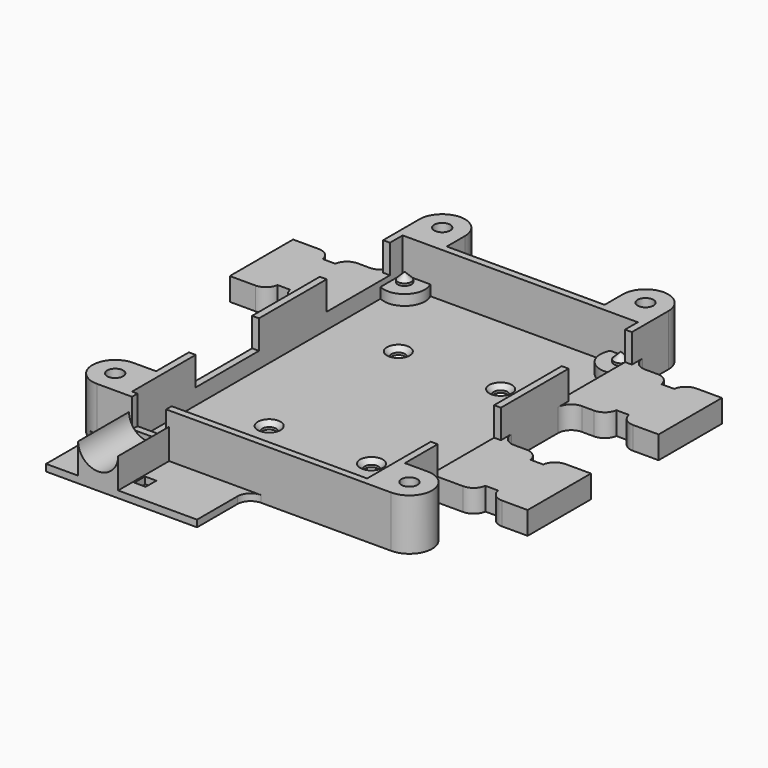
from build123d import *

# Parameters (mm, degrees)
F1_W          = 54.708
F1_H          = 77.4
F2_DEPTH      = 11.3
F3_T          = -1.5
F4_W          = 20.1
F4_H          = 17.4
F5_DEPTH      = 6.3
F6_R          = 4.5
F7_DEPTH      = 2.3
F8_R          = 1.5
F9_DEPTH      = 11.301
F10_SIZE      = 1
F11_R         = 1.75
F12_DEPTH     = 11.3
F13_R         = 1.5
F14_DEPTH     = 2
F15_SIZE      = 1.5
F16_W         = 7.5
F16_H         = 1.5
F17_DEPTH     = 6.3
F18_W         = 19.8
F18_H         = 17.4
F19_DEPTH     = 5
F20_W         = 33.2
F20_H         = 14
F21_DEPTH     = 1.5
F23_DEPTH     = 14
F24_W         = 2.5
F24_H         = 2.8
F24_W_2       = 2.8
F24_H_2       = 2.5
F24_W_3       = 2.5000000001
F24_H_3       = 2.940192353
F25_DEPTH     = 11.301
F26_T1_DEPTH  = 1.5
F26_T3_DEPTH  = 1.5
F26_T5_DEPTH  = 5
F26_T7_DEPTH  = 5
F26_T9_DEPTH  = 5
F26_T11_DEPTH = 5
F26_T13_DEPTH = 5
F26_T15_DEPTH = 19.3614066163
F26_T17_DEPTH = 19.3614066163
F26_T19_DEPTH = 19.3614066163
F26_T21_DEPTH = 19.3614066163
F26_T23_DEPTH = 19.3614066163
F26_T25_DEPTH = 19.3614066163
F26_T27_DEPTH = 19.3614066163
F26_T29_DEPTH = 19.3614066163
F26_T31_DEPTH = 19.3614066163
F26_T33_DEPTH = 19.3614066163
F26_T35_DEPTH = 19.3614066163
F26_T37_DEPTH = 19.3614066163


# Not quite as in the source:
# - a fillet or chamfer that OpenCascade refuses, or shapes differently, is made with other operations: its cross-section is extruded or revolved along the edge and cut away or added


with BuildPart() as f2:
    # F1 (on face) → F2 (new body)
    with BuildSketch(Plane.XY):
        with Locations((25.654, 37)):
            Rectangle(F1_W, F1_H)
    extrude(amount=F2_DEPTH)

    # F3
    f3_openings = [f2.faces().sort_by_distance(p)[0] for p in [
        (25.654, 37, 11.3),
    ]]
    offset(amount=F3_T, openings=f3_openings)

    # F4 (on face) → F5 (cut, through all)
    with BuildSketch(Plane.XY.offset(11.3)):
        with Locations((8.35, 26)):
            Rectangle(F4_W, F4_H)
        with Locations((42.958, 26)):
            Rectangle(F4_W, F4_H)
        with Locations((8.35, 62)):
            Rectangle(F4_W, F4_H)
        with Locations((42.958, 62)):
            Rectangle(F4_W, F4_H)
    extrude(amount=-F5_DEPTH, mode=Mode.SUBTRACT)

    # F6 (on face) → F7 (join, through all)
    with BuildSketch(Plane.XY.offset(1.5)):
        with BuildLine():
            Line((-1.7, 74.8469880528), (-1.7, 69.3930119472))
            ThreePointArc((-1.7, 69.3930119472), (6.3796, 72.12), (-1.7, 74.8469880528))
        make_face()
        with BuildLine():
            Line((53.008, 69.3930119472), (53.008, 74.8469880528))
            ThreePointArc((53.008, 74.8469880528), (44.9284, 72.12), (53.008, 69.3930119472))
        make_face()
        with Locations((11.2141, 3.9243)):
            Circle(F6_R)
        with Locations((32.512, 3.9243)):
            Circle(F6_R)
        with BuildLine():
            Line((53.008, 1.1973119472), (53.008, 6.6512880528))
            ThreePointArc((53.008, 6.6512880528), (44.9284, 3.9243), (53.008, 1.1973119472))
        make_face()
    extrude(amount=F7_DEPTH)

    # F8 (on face) → F9 (cut, through all)
    with BuildSketch(Plane(origin=(0, 0, 0), x_dir=(1, 0, 0), z_dir=(0, 0, -1))):
        with Locations((14.404, -54.75)):
            Circle(F8_R)
        with Locations((14.404, -19.25)):
            Circle(F8_R)
        with Locations((36.904, -19.25)):
            Circle(F8_R)
        with Locations((36.904, -54.75)):
            Circle(F8_R)
    extrude(amount=-F9_DEPTH, mode=Mode.SUBTRACT)

    # F10
    f10_edges = [f2.edges().sort_by_distance(p)[0] for p in [
        (35.404, 54.75, 1.5),
        (12.904, 54.75, 1.5),
        (35.404, 19.25, 1.5),
        (12.904, 19.25, 1.5),
    ]]
    chamfer(f10_edges, length=F10_SIZE)

    # F11 (on face) → F12 (join, through all)
    with BuildSketch(Plane(origin=(0, 0, 0), x_dir=(1, 0, 0), z_dir=(0, 0, -1))):
        with BuildLine():
            Line((-1.7, 1.7), (-6.7, 1.7))
            ThreePointArc((-6.7, 1.7), (-11.7, -3.3), (-6.7, -8.3))
            Line((-6.7, -8.3), (-1.7, -8.3))
            Line((-1.7, -8.3), (-1.7, 1.7))
        make_face()
        with Locations((-6.7, -3.3)):
            Circle(F11_R, mode=Mode.SUBTRACT)
        with BuildLine():
            Line((-1.7, -75.7), (-1.7, -80.7))
            ThreePointArc((-1.7, -80.7), (3.3, -85.7), (8.3, -80.7))
            Line((8.3, -80.7), (8.3, -75.7))
            Line((8.3, -75.7), (-1.7, -75.7))
        make_face()
        with Locations((3.3, -80.7)):
            Circle(F11_R, mode=Mode.SUBTRACT)
        with BuildLine():
            Line((53.008, -8.3), (58.008, -8.3))
            ThreePointArc((58.008, -8.3), (63.008, -3.3), (58.008, 1.7))
            Line((58.008, 1.7), (53.008, 1.7))
            Line((53.008, 1.7), (53.008, -8.3))
        make_face()
        with Locations((58.008, -3.3)):
            Circle(F11_R, mode=Mode.SUBTRACT)
        with BuildLine():
            Line((43.008, -75.7), (43.008, -80.7))
            ThreePointArc((43.008, -80.7), (48.008, -85.7), (53.008, -80.7))
            Line((53.008, -80.7), (53.008, -75.7))
            Line((53.008, -75.7), (43.008, -75.7))
        make_face()
        with Locations((48.008, -80.7)):
            Circle(F11_R, mode=Mode.SUBTRACT)
    extrude(amount=-F12_DEPTH)

    # F13 (on face) → F14 (join)
    with BuildSketch(Plane.XY.offset(3.8)):
        with Locations((49.4284, 3.9243)):
            Circle(F13_R)
        with Locations((32.512, 3.9243)):
            Circle(F13_R)
        with Locations((11.2141, 3.9243)):
            Circle(F13_R)
        with Locations((49.4284, 72.12)):
            Circle(F13_R)
        with Locations((1.8796, 72.12)):
            Circle(F13_R)
    extrude(amount=F14_DEPTH)

    # F15
    f15_edges = [f2.edges().sort_by_distance(p)[0] for p in [
        (47.9284, 3.9243, 5.8),
        (31.012, 3.9243, 5.8),
        (9.7141, 3.9243, 5.8),
        (47.9284, 72.12, 5.8),
        (0.3796, 72.12, 5.8),
    ]]
    chamfer(f15_edges, length=F15_SIZE)

    # F16 (on face) → F17 (cut, through all)
    with BuildSketch(Plane.XY.offset(11.3)):
        with Locations((4.75, -0.95)):
            Rectangle(F16_W, F16_H)
    extrude(amount=-F17_DEPTH, mode=Mode.SUBTRACT)

    # F18 (on face) → F19 (join, through all)
    with BuildSketch(Plane(origin=(0, 0, 0), x_dir=(1, 0, 0), z_dir=(0, 0, -1))):
        with Locations((-11.6, -62)):
            Rectangle(F18_W, F18_H)
        with Locations((62.908, -62)):
            Rectangle(F18_W, F18_H)
        with Locations((62.908, -26)):
            Rectangle(F18_W, F18_H)
    extrude(amount=-F19_DEPTH)

    # F20 (on face) → F21 (join)
    with BuildSketch(Plane(origin=(0, 0, 0), x_dir=(1, 0, 0), z_dir=(0, 0, -1))):
        with Locations((9.9, 8.7)):
            Rectangle(F20_W, F20_H)
    extrude(amount=-F21_DEPTH)

    # F22 (on face) → F23 (join, through all)
    with BuildSketch(Plane.XZ.offset(1.7)):
        with BuildLine():
            ThreePointArc((9.15, 8.1499999998), (4.75, 3.7499999995), (0.35, 8.1499999998))
            Line((0.35, 8.1499999998), (0.35, 1.5))
            Line((0.35, 1.5), (9.15, 1.5))
            Line((9.15, 1.5), (9.15, 8.1499999998))
        make_face()
    extrude(amount=F23_DEPTH)

    # F24 (on face) → F25 (cut, through all)
    with BuildSketch(Plane(origin=(0, 0, 0), x_dir=(1, 0, 0), z_dir=(0, 0, -1))):
        with Locations((-0.9, 10.3)):
            Rectangle(F24_W, F24_H)
        with Locations((-11.6, -54.55)):
            Rectangle(F24_W_2, F24_H_2)
        with Locations((10.7548580677, 10.2299038235)):
            Rectangle(F24_W_3, F24_H_3)
        with Locations((-11.6, -69.45)):
            Rectangle(F24_W_2, F24_H_2)
        with Locations((62.908, -69.45)):
            Rectangle(F24_W_2, F24_H_2)
        with Locations((62.908, -54.55)):
            Rectangle(F24_W_2, F24_H_2)
        with Locations((62.908, -18.55)):
            Rectangle(F24_W_2, F24_H_2)
        with Locations((62.908, -33.45)):
            Rectangle(F24_W_2, F24_H_2)
    extrude(amount=-F25_DEPTH, mode=Mode.SUBTRACT)

    # F26: fillet of radius 2.9 on 20 edges, made by hand

    # F26_s2 → F26_t1 (join)
    with BuildSketch(Plane.XY):
        with BuildLine():
            ThreePointArc((-8.535443038, -1.3509298914), (-7.2023745924, -2.417091772), (-6.7, -4.0484692283))
            Line((-6.7, -4.0484692283), (-6.7, -1.7))
            ThreePointArc((-6.7, -1.7), (-7.6341709006, -1.6119573215), (-8.535443038, -1.3509298914))
        make_face()
    extrude(amount=F26_T1_DEPTH)

    # F26_s4 → F26_t3 (join)
    with BuildSketch(Plane.XY):
        with BuildLine():
            ThreePointArc((29.4, -1.7), (27.3493903346, -2.5493903346), (26.5, -4.6))
            Line((26.5, -4.6), (26.5, -1.7))
            Line((26.5, -1.7), (29.4, -1.7))
        make_face()
    extrude(amount=F26_T3_DEPTH)

    # F26_s6 → F26_t5 (join)
    with BuildSketch(Plane.XY):
        with BuildLine():
            ThreePointArc((53.008, 37.6), (53.8573903346, 35.5493903346), (55.908, 34.7))
            Line((55.908, 34.7), (53.008, 34.7))
            Line((53.008, 34.7), (53.008, 37.6))
        make_face()
    extrude(amount=F26_T5_DEPTH)

    # F26_s8 → F26_t7 (join)
    with BuildSketch(Plane.XY):
        with BuildLine():
            ThreePointArc((55.908, 53.3), (53.8573903346, 52.4506096654), (53.008, 50.4))
            Line((53.008, 50.4), (53.008, 53.3))
            Line((53.008, 53.3), (55.908, 53.3))
        make_face()
    extrude(amount=F26_T7_DEPTH)

    # F26_s10 → F26_t9 (join)
    with BuildSketch(Plane.XY):
        with BuildLine():
            ThreePointArc((53.008, 73.6), (53.8573903346, 71.5493903346), (55.908, 70.7))
            Line((55.908, 70.7), (53.008, 70.7))
            Line((53.008, 70.7), (53.008, 73.6))
        make_face()
    extrude(amount=F26_T9_DEPTH)

    # F26_s12 → F26_t11 (join)
    with BuildSketch(Plane.XY):
        with BuildLine():
            ThreePointArc((-4.6, 70.7), (-2.5493903346, 71.5493903346), (-1.7, 73.6))
            Line((-1.7, 73.6), (-1.7, 70.7))
            Line((-1.7, 70.7), (-4.6, 70.7))
        make_face()
    extrude(amount=F26_T11_DEPTH)

    # F26_s14 → F26_t13 (join)
    with BuildSketch(Plane.XY):
        with BuildLine():
            ThreePointArc((-1.7, 50.4), (-2.5493903346, 52.4506096654), (-4.6, 53.3))
            Line((-4.6, 53.3), (-1.7, 53.3))
            Line((-1.7, 53.3), (-1.7, 50.4))
        make_face()
    extrude(amount=F26_T13_DEPTH)

    # F26_s16 → F26_t15 (cut)
    with BuildSketch(Plane.XY.offset(-7.1807033082)):
        with BuildLine():
            ThreePointArc((58.6357186767, 17.3), (60.5396619532, 18.0125357146), (61.508, 19.8))
            Line((61.508, 19.8), (61.508, 17.3))
            Line((61.508, 17.3), (58.6357186767, 17.3))
        make_face()
    extrude(amount=F26_T15_DEPTH, mode=Mode.SUBTRACT)

    # F26_s18 → F26_t17 (cut)
    with BuildSketch(Plane.XY.offset(-7.1807033082)):
        with BuildLine():
            ThreePointArc((67.1802813233, 17.3), (65.2763380468, 18.0125357146), (64.308, 19.8))
            Line((64.308, 19.8), (64.308, 17.3))
            Line((64.308, 17.3), (67.1802813233, 17.3))
        make_face()
    extrude(amount=F26_T17_DEPTH, mode=Mode.SUBTRACT)

    # F26_s20 → F26_t19 (cut)
    with BuildSketch(Plane.XY.offset(-7.1807033082)):
        with BuildLine():
            ThreePointArc((64.308, 32.2), (65.2763380468, 33.9874642854), (67.1802813233, 34.7))
            Line((67.1802813233, 34.7), (64.308, 34.7))
            Line((64.308, 34.7), (64.308, 32.2))
        make_face()
    extrude(amount=F26_T19_DEPTH, mode=Mode.SUBTRACT)

    # F26_s22 → F26_t21 (cut)
    with BuildSketch(Plane.XY.offset(-7.1807033082)):
        with BuildLine():
            ThreePointArc((58.6357186767, 34.7), (60.5396619532, 33.9874642854), (61.508, 32.2))
            Line((61.508, 32.2), (61.508, 34.7))
            Line((61.508, 34.7), (58.6357186767, 34.7))
        make_face()
    extrude(amount=F26_T21_DEPTH, mode=Mode.SUBTRACT)

    # F26_s24 → F26_t23 (cut)
    with BuildSketch(Plane.XY.offset(-7.1807033082)):
        with BuildLine():
            ThreePointArc((58.6357186767, 53.3), (60.5396619532, 54.0125357146), (61.508, 55.8))
            Line((61.508, 55.8), (61.508, 53.3))
            Line((61.508, 53.3), (58.6357186767, 53.3))
        make_face()
    extrude(amount=F26_T23_DEPTH, mode=Mode.SUBTRACT)

    # F26_s26 → F26_t25 (cut)
    with BuildSketch(Plane.XY.offset(-7.1807033082)):
        with BuildLine():
            ThreePointArc((67.1802813233, 53.3), (65.2763380468, 54.0125357146), (64.308, 55.8))
            Line((64.308, 55.8), (64.308, 53.3))
            Line((64.308, 53.3), (67.1802813233, 53.3))
        make_face()
    extrude(amount=F26_T25_DEPTH, mode=Mode.SUBTRACT)

    # F26_s28 → F26_t27 (cut)
    with BuildSketch(Plane.XY.offset(-7.1807033082)):
        with BuildLine():
            ThreePointArc((64.308, 68.2), (65.2763380468, 69.9874642854), (67.1802813233, 70.7))
            Line((67.1802813233, 70.7), (64.308, 70.7))
            Line((64.308, 70.7), (64.308, 68.2))
        make_face()
    extrude(amount=F26_T27_DEPTH, mode=Mode.SUBTRACT)

    # F26_s30 → F26_t29 (cut)
    with BuildSketch(Plane.XY.offset(-7.1807033082)):
        with BuildLine():
            ThreePointArc((58.6357186767, 70.7), (60.5396619532, 69.9874642854), (61.508, 68.2))
            Line((61.508, 68.2), (61.508, 70.7))
            Line((61.508, 70.7), (58.6357186767, 70.7))
        make_face()
    extrude(amount=F26_T29_DEPTH, mode=Mode.SUBTRACT)

    # F26_s32 → F26_t31 (cut)
    with BuildSketch(Plane.XY.offset(-7.1807033082)):
        with BuildLine():
            ThreePointArc((-7.3277186767, 70.7), (-9.2316619532, 69.9874642854), (-10.2, 68.2))
            Line((-10.2, 68.2), (-10.2, 70.7))
            Line((-10.2, 70.7), (-7.3277186767, 70.7))
        make_face()
    extrude(amount=F26_T31_DEPTH, mode=Mode.SUBTRACT)

    # F26_s34 → F26_t33 (cut)
    with BuildSketch(Plane.XY.offset(-7.1807033082)):
        with BuildLine():
            ThreePointArc((-15.8722813233, 70.7), (-13.9683380468, 69.9874642854), (-13, 68.2))
            Line((-13, 68.2), (-13, 70.7))
            Line((-13, 70.7), (-15.8722813233, 70.7))
        make_face()
    extrude(amount=F26_T33_DEPTH, mode=Mode.SUBTRACT)

    # F26_s36 → F26_t35 (cut)
    with BuildSketch(Plane.XY.offset(-7.1807033082)):
        with BuildLine():
            ThreePointArc((-13, 55.8), (-13.9683380468, 54.0125357146), (-15.8722813233, 53.3))
            Line((-15.8722813233, 53.3), (-13, 53.3))
            Line((-13, 53.3), (-13, 55.8))
        make_face()
    extrude(amount=F26_T35_DEPTH, mode=Mode.SUBTRACT)

    # F26_s38 → F26_t37 (cut)
    with BuildSketch(Plane.XY.offset(-7.1807033082)):
        with BuildLine():
            ThreePointArc((-7.3277186767, 53.3), (-9.2316619532, 54.0125357146), (-10.2, 55.8))
            Line((-10.2, 55.8), (-10.2, 53.3))
            Line((-10.2, 53.3), (-7.3277186767, 53.3))
        make_face()
    extrude(amount=F26_T37_DEPTH, mode=Mode.SUBTRACT)


solid = f2.part
